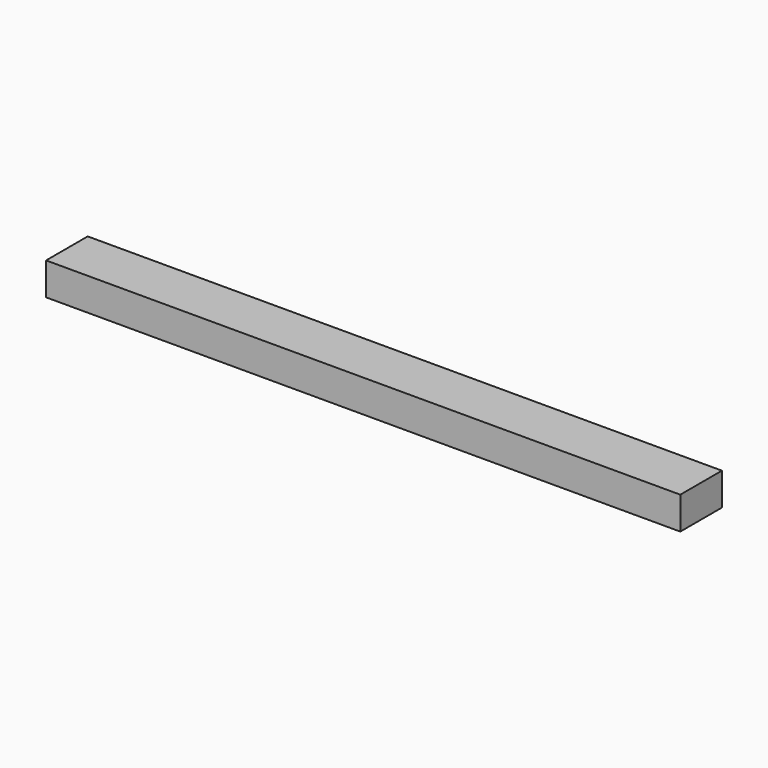
from build123d import *

# Parameters (mm, degrees)
F0_W     = 406.4
F0_H     = 254
F1_DEPTH = 4953


with BuildPart() as f1:
    # F0 (on Right) → F1 (new body)
    with BuildSketch(Plane.YZ):
        Rectangle(F0_W, F0_H)
    extrude(amount=F1_DEPTH)


solid = f1.part
